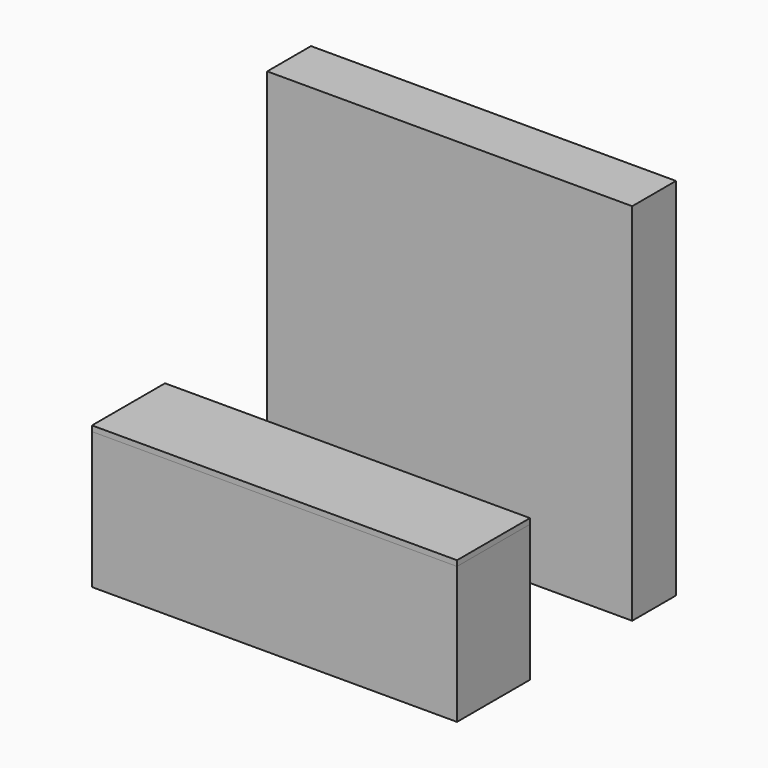
from build123d import *

# Parameters (mm, degrees)
F1_W     = 2000
F1_H     = 300
F2_DEPTH = 2000
F4_DEPTH = 750
F5_W     = 2000
F5_H     = 500
F6_DEPTH = 30


with BuildPart() as f2:
    # F1 (on Top) → F2 (new body)
    with BuildSketch(Plane.XY):
        with Locations((0, 600)):
            Rectangle(F1_W, F1_H)
    extrude(amount=F2_DEPTH)


with BuildPart() as f4:
    # F3 (on Top) → F4 (new body)
    with BuildSketch(Plane.XY):
        Polygon((1000, -750), (1000, -250), (970, -250), (970, -720), (-970, -720), (-970, -250), (-1000, -250), (-1000, -750), align=None)
    extrude(amount=F4_DEPTH)


with BuildPart() as f6:
    # F5 (on face) → F6 (new body)
    with BuildSketch(Plane.XY.offset(750)):
        with Locations((0, -500)):
            Rectangle(F5_W, F5_H)
    extrude(amount=F6_DEPTH)


with BuildPart() as f7_1:
    # F7: instance of F2
    add(f2.part.mirror(Plane.YZ))


solid = Compound([f2.part, f4.part, f6.part])
